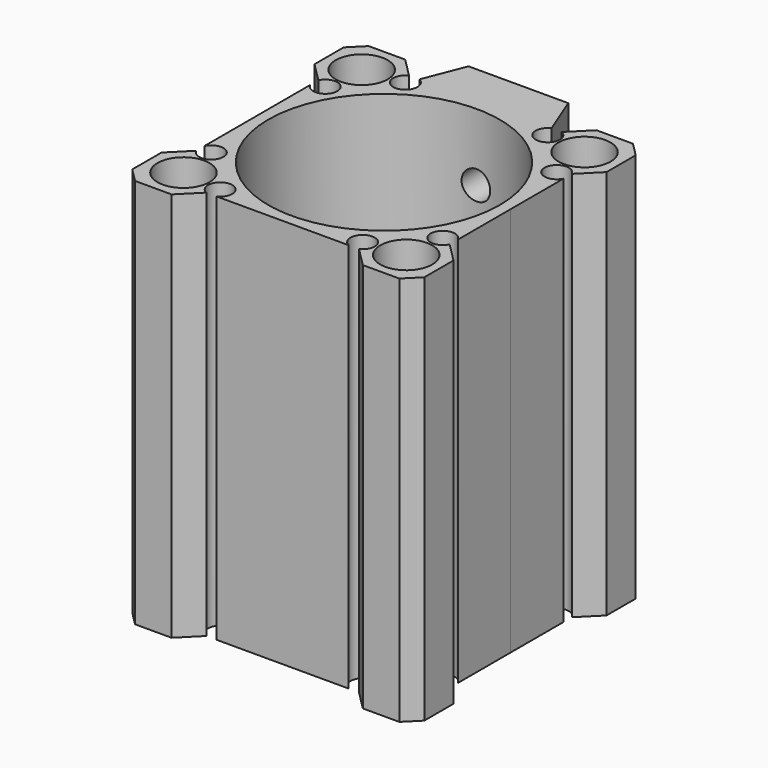
from build123d import *

# Parameters (mm, degrees)
F0_R           = 4.6355
F1_DEPTH       = 69.596
F2_D           = 5.588
F2_CBORE_D     = 9.271
F2_CBORE_DEPTH = 7.366
F3_D           = 41.275
F5_D           = 5.1054
F5_DEPTH       = 16.51
F5_TIP         = 1.5338169022


# Not quite as in the source:
# - ends of sketch curves that miss each other by under 0.0002 mm in the source are joined


with BuildPart() as f1:
    # F0 (on Top) → F1 (new body)
    with BuildSketch(Plane.XY):
        with BuildLine():
            Line((0, 20.828), (0, 22.5937319184))
            Line((0, 22.5937319184), (-11.7865243948, 22.593731583))
            ThreePointArc((-11.7865243948, 22.593731583), (-12.6999991591, 18.4785002754), (-13.613476896, 22.593731531))
            Line((-13.613476896, 22.593731531), (-17.0547434947, 26.035))
            Line((-17.0547434947, 26.035), (-23.5585, 26.035))
            Line((-23.5585, 26.035), (-26.035, 23.5585))
            Line((-26.035, 23.5585), (-26.035, 17.0547438789))
            Line((-26.035, 17.0547438789), (-22.5937318573, 13.6134757362))
            ThreePointArc((-22.5937318573, 13.6134757362), (-18.4785, 12.7), (-22.5937318573, 11.7865242638))
            Line((-22.5937318573, 11.7865242638), (-22.5937318573, -11.7865242638))
            ThreePointArc((-22.5937318573, -11.7865242638), (-18.4785, -12.7), (-22.5937318573, -13.6134757362))
            Line((-22.5937318573, -13.6134757362), (-26.035, -17.0547438789))
            Line((-26.035, -17.0547438789), (-26.035, -23.5585))
            Line((-26.035, -23.5585), (-23.5585, -26.035))
            Line((-23.5585, -26.035), (-17.0547438789, -26.035))
            Line((-17.0547438789, -26.035), (-13.6134757362, -22.5937318573))
            ThreePointArc((-13.6134757362, -22.5937318573), (-12.7, -18.4785), (-11.7865242638, -22.5937318573))
            Line((-11.7865242638, -22.5937318573), (11.7865242638, -22.5937318573))
            ThreePointArc((11.7865242638, -22.5937318573), (12.7, -18.4785), (13.6134757362, -22.5937318573))
            Line((13.6134757362, -22.5937318573), (17.0547438789, -26.035))
            Line((17.0547438789, -26.035), (23.5585, -26.035))
            Line((23.5585, -26.035), (26.035, -23.5585))
            Line((26.035, -23.5585), (26.035, -17.0547434947))
            Line((26.035, -17.0547434947), (22.5937319796, -13.6134754743))
            ThreePointArc((22.5937319796, -13.6134754743), (18.4785, -12.7000000097), (22.5937319714, -11.7865245082))
            Line((22.5937319714, -11.7865245082), (22.5937319184, 0))
            Line((22.5937319184, 0), (20.828, 0))
            ThreePointArc((20.828, 0), (-14.7276200386, -14.7276200386), (0, 20.828))
        make_face()
        with Locations((-19.8628, -19.8628)):
            Circle(F0_R, mode=Mode.SUBTRACT)
        with Locations((19.8628, -19.8628)):
            Circle(F0_R, mode=Mode.SUBTRACT)
        with Locations((-19.8628, 19.8628)):
            Circle(F0_R, mode=Mode.SUBTRACT)
        Polygon((0, 22.5937319184), (11.7865243948, 22.5937322538), (8.8899997904, 29.9597321714), (-8.89, 29.9597316654), (-11.7865243948, 22.593731583), align=None)
        with BuildLine():
            Line((26.035, 23.5585), (23.5585, 26.035))
            Line((23.5585, 26.035), (17.0547438789, 26.035))
            Line((17.0547438789, 26.035), (13.6134752367, 22.5937323058))
            ThreePointArc((13.6134752367, 22.5937323058), (12.6999999329, 18.4785002754), (11.7865243948, 22.5937322538))
            Line((11.7865243948, 22.5937322538), (0, 22.5937319184))
            Line((0, 22.5937319184), (0, 20.828))
            ThreePointArc((0, 20.828), (14.7276200386, 14.7276200386), (20.828, 0))
            Line((20.828, 0), (22.5937319184, 0))
            Line((22.5937319184, 0), (22.5937318655, 11.7865242814))
            ThreePointArc((22.5937318655, 11.7865242814), (18.4785, 12.6999999903), (22.5937318573, 13.6134757362))
            Line((22.5937318573, 13.6134757362), (26.035, 17.0547438789))
            Line((26.035, 17.0547438789), (26.035, 23.5585))
        make_face()
        with Locations((19.8628, 19.8628)):
            Circle(F0_R, mode=Mode.SUBTRACT)
        with Locations((19.8628, -19.8628)):
            Circle(F0_R)
        with Locations((19.8628, 19.8628)):
            Circle(F0_R)
        with Locations((-19.8628, 19.8628)):
            Circle(F0_R)
        with Locations((-19.8628, -19.8628)):
            Circle(F0_R)
        with BuildLine():
            ThreePointArc((20.828, 0), (14.7276200386, 14.7276200386), (0, 20.828))
            Line((0, 20.828), (0, 0))
            Line((0, 0), (20.828, 0))
        make_face()
        with BuildLine():
            Line((0, 0), (0, 20.828))
            ThreePointArc((0, 20.828), (-14.7276200386, -14.7276200386), (20.828, 0))
            Line((20.828, 0), (0, 0))
        make_face()
    extrude(amount=-F1_DEPTH)

    # F2 (through all)
    with Locations(Plane.XY):
        with Locations((-19.8628, 19.8628), (19.8628, 19.8628), (19.8628, -19.8628), (-19.8628, -19.8628)):
            CounterBoreHole(F2_D / 2, F2_CBORE_D / 2, F2_CBORE_DEPTH)

    # F3 (through all)
    with Locations(Plane.XY):
        with Locations((0, 0)):
            Hole(F3_D / 2)

    # F5
    with Locations(Plane(origin=(-8.526e-07, 29.9597319184, 0), x_dir=(-1, -2.85e-08, 0), z_dir=(-2.85e-08, 1, 0))):
        with Locations((0, -11.9891270243), (0, -53.7712314358)):
            Hole(F5_D / 2, depth=F5_DEPTH)
            with Locations((0, 0, -(F5_DEPTH + F5_TIP / 2))):  # 118° drill point
                Cone(0, F5_D / 2, F5_TIP, mode=Mode.SUBTRACT)


solid = f1.part
